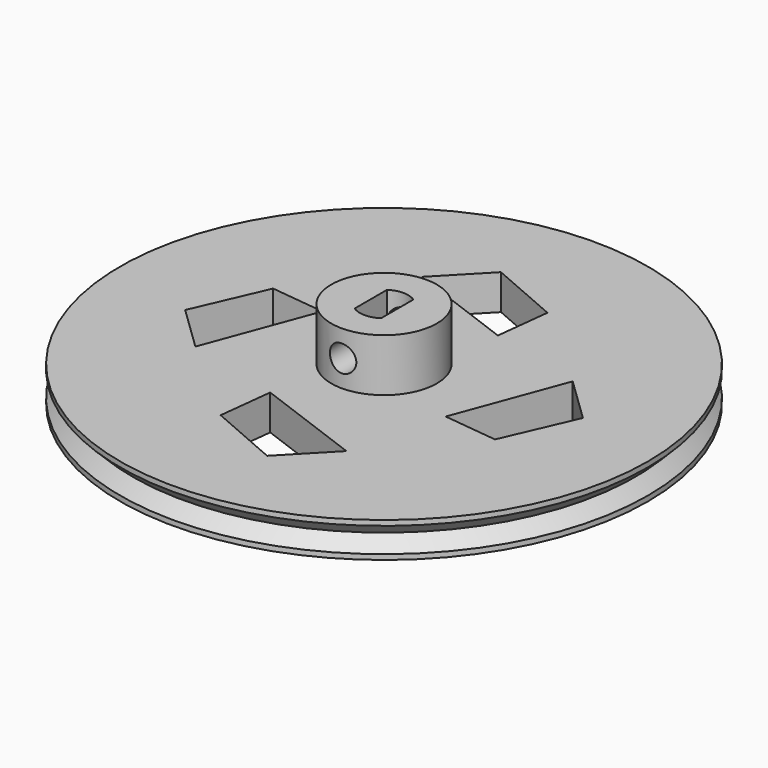
from build123d import *

# Parameters (mm, degrees)
F0_R             = 30
F0_R_2           = 6
F1_DEPTH         = 4
F2_DEPTH         = 6
F3_R             = 1.5
F4_DEPTH         = 12.5
F5_W             = 3
F5_H             = 4.6
F6_DEPTH         = 9.4
F10_DEPTH        = 4
F10_COPIES_COUNT = 4


# Not quite as in the source:
# - a pattern or mirror of a feature is missing from the dataset's text; its kind, count and spacing are read off the source's solid


with BuildPart() as f1:
    # F0 (on Top) → F1 (new body)
    with BuildSketch(Plane.XY):
        Circle(F0_R)
        Circle(F0_R_2, mode=Mode.SUBTRACT)
    extrude(amount=-F1_DEPTH)

    # F7 (on Front) → F8 (revolve, cut)
    with BuildSketch(Plane.XZ):
        Polygon((-30, -0.5857864376), (-30, -3.4142135624), (-28.5857864376, -2), align=None)
    revolve(axis=Axis((0, 0, 1.4569712803), (0, 0, -1)), mode=Mode.SUBTRACT)

    # F9 (on face) → F10 (cut, through all)
    with BuildSketch(Plane.XY):
        Polygon((-2.9223964084, 20.2681515366), (-7.8513491899, 15.1631673798), (4.471027758, 10.586284101), (5.1751635037, 16.7474728078), align=None)
    f10 = extrude(amount=-F10_DEPTH, mode=Mode.SUBTRACT)

    # F10_copies: F10 ×4 about axis
    f10_copies_axis = Axis((0, 0, 0), (0, 0, 1))
    for i in range(1, F10_COPIES_COUNT):
        add(f10.rotate(f10_copies_axis, i * 360 / F10_COPIES_COUNT), mode=Mode.SUBTRACT)


with BuildPart() as f2:
    # F0 (on Top) → F2 (new body)
    with BuildSketch(Plane.XY):
        Circle(F0_R_2)
    extrude(amount=F2_DEPTH)

    # F3 (on Front) → F4 (cut, symmetric)
    with BuildSketch(Plane.XZ):
        with Locations((0, 3)):
            Circle(F3_R)
    extrude(amount=F4_DEPTH, both=True, mode=Mode.SUBTRACT)

    # F5 (on face) → F6 (cut)
    with BuildSketch(Plane.XY.offset(6)):
        Rectangle(F5_W, F5_H)
        with BuildLine():
            Line((1.5, -2.3), (-1.5, -2.3))
            ThreePointArc((-1.5, -2.3), (0, -2.7540939565), (1.5, -2.3))
        make_face()
        with BuildLine():
            ThreePointArc((1.5, 2.3), (0, 2.7459060435), (-1.5, 2.3))
            Line((-1.5, 2.3), (1.5, 2.3))
        make_face()
    extrude(amount=-F6_DEPTH, mode=Mode.SUBTRACT)


solid = Compound([f1.part, f2.part])
